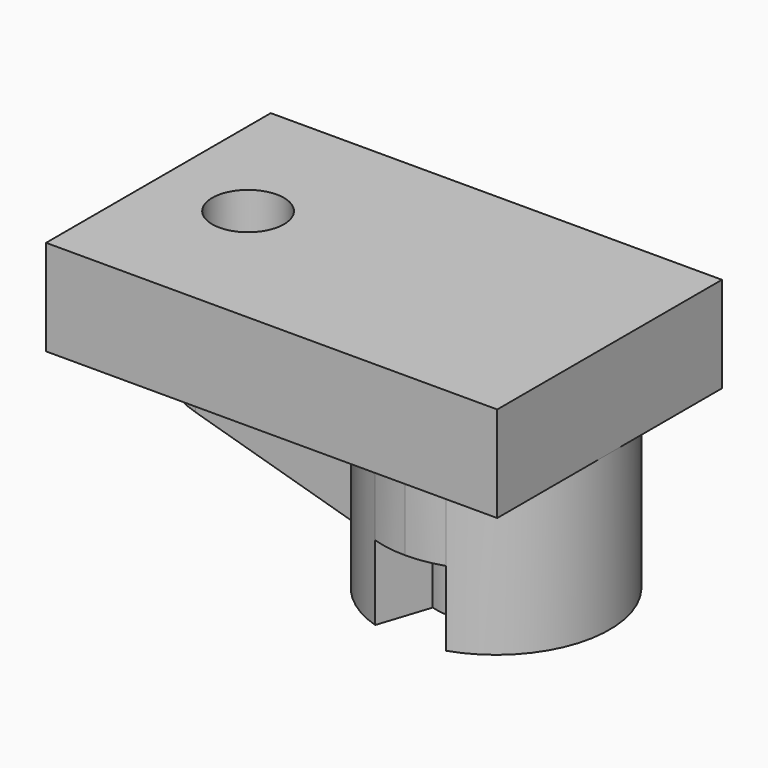
from build123d import *

# Parameters (mm, degrees)
F0_R      = 12
F1_DEPTH  = 32
F2_DEPTH  = 12
F3_DEPTH  = 52
F5_DEPTH  = 44
F6_DEPTH  = 93.7
F7_R      = 12
F8_DEPTH  = 98.4
F9_DEPTH  = 52
F11_DEPTH = 25


# Not quite as in the source:
# - a feature names something its author has since deleted; it is built from what else it names


with BuildPart() as f1:
    # F0 (on Top) → F1 (new body)
    with BuildSketch(Plane.XY):
        with BuildLine():
            Line((35.3547130823, 81.2151380405), (-47.6452869177, 81.2151380405))
            Line((-47.6452869177, 81.2151380405), (-47.6452869177, 56.2151380405))
            Line((-47.6452869177, 56.2151380405), (4.3708463127, 56.2151380405))
            ThreePointArc((4.3708463127, 56.2151380405), (13.0601260183, 64.9877132925), (24.1033321201, 70.5112318584))
            ThreePointArc((24.1033321201, 70.5112318584), (29.6648785101, 71.7867467702), (35.3547130823, 72.2151380405))
            Line((35.3547130823, 72.2151380405), (35.3547130823, 81.2151380405))
        make_face()
        with BuildLine():
            Line((-47.6452869177, 81.2151380405), (-77.6452869177, 81.2151380405))
            Line((-77.6452869177, 81.2151380405), (-77.6452869177, -12.7848619595))
            Line((-77.6452869177, -12.7848619595), (-47.6452869177, -12.7848619595))
            Line((-47.6452869177, -12.7848619595), (35.3547130823, -12.7848619595))
            Line((35.3547130823, -12.7848619595), (35.3547130823, -3.7848619595))
            ThreePointArc((35.3547130823, -3.7848619595), (29.5441458382, -3.3379884379), (23.8702411544, -2.0078781859))
            ThreePointArc((23.8702411544, -2.0078781859), (12.9613324626, 3.5143806488), (4.3708463127, 12.2151380405))
            Line((4.3708463127, 12.2151380405), (-47.6452869177, 12.2151380405))
            ThreePointArc((-47.6452869177, 12.2151380405), (-69.6452869177, 34.2151380405), (-47.6452869177, 56.2151380405))
            Line((-47.6452869177, 56.2151380405), (-47.6452869177, 81.2151380405))
        make_face()
        with BuildLine():
            Line((4.3708463127, 56.2151380405), (-47.6452869177, 56.2151380405))
            ThreePointArc((-47.6452869177, 56.2151380405), (-32.0889377316, 49.7714872266), (-25.6452869177, 34.2151380405))
            Line((-25.6452869177, 34.2151380405), (-2.6452869177, 34.2151380405))
            ThreePointArc((-2.6452869177, 34.2151380405), (-0.8487876963, 45.7609828072), (4.3708463127, 56.2151380405))
        make_face()
        with BuildLine():
            Line((-2.6452869177, 34.2151380405), (-25.6452869177, 34.2151380405))
            ThreePointArc((-25.6452869177, 34.2151380405), (-32.0889377316, 18.6587888544), (-47.6452869177, 12.2151380405))
            Line((-47.6452869177, 12.2151380405), (4.3708463127, 12.2151380405))
            ThreePointArc((4.3708463127, 12.2151380405), (-0.8487876963, 22.6692932738), (-2.6452869177, 34.2151380405))
        make_face()
        with BuildLine():
            ThreePointArc((-25.6452869177, 34.2151380405), (-32.0889377316, 49.7714872266), (-47.6452869177, 56.2151380405))
            ThreePointArc((-47.6452869177, 56.2151380405), (-69.6452869177, 34.2151380405), (-47.6452869177, 12.2151380405))
            ThreePointArc((-47.6452869177, 12.2151380405), (-32.0889377316, 18.6587888544), (-25.6452869177, 34.2151380405))
        make_face()
        with Locations((-47.6452869177, 34.2151380405)):
            Circle(F0_R, mode=Mode.SUBTRACT)
        with Locations((-47.6452869177, 34.2151380405)):
            Circle(F0_R)
        with BuildLine():
            ThreePointArc((24.1033321201, 70.5112318584), (13.0601260183, 64.9877132925), (4.3708463127, 56.2151380405))
            ThreePointArc((4.3708463127, 56.2151380405), (-0.8487876963, 45.7609828072), (-2.6452869177, 34.2151380405))
            ThreePointArc((-2.6452869177, 34.2151380405), (-0.8487876963, 22.6692932738), (4.3708463127, 12.2151380405))
            ThreePointArc((4.3708463127, 12.2151380405), (12.9613324626, 3.5143806488), (23.8702411544, -2.0078781859))
            Line((23.8702411544, -2.0078781859), (29.4328161154, 15.111967196))
            ThreePointArc((29.4328161154, 15.111967196), (32.3600024861, 14.440616341), (35.3547130823, 14.2151380405))
            Line((35.3547130823, 14.2151380405), (35.3547130823, 54.2151380405))
            ThreePointArc((35.3547130823, 54.2151380405), (32.4808372386, 54.0075819935), (29.6666104259, 53.389221804))
            Line((29.6666104259, 53.389221804), (24.1033321201, 70.5112318584))
        make_face()
        with BuildLine():
            ThreePointArc((47.4336065252, -1.8140214445), (66.2010901048, 12.0227739351), (73.3547130823, 34.2151380405))
            ThreePointArc((73.3547130823, 34.2151380405), (66.1022036315, 56.5443078622), (47.1130380862, 70.3501874123))
            Line((47.1130380862, 70.3501874123), (41.5507311927, 53.2311670575))
            ThreePointArc((41.5507311927, 53.2311670575), (38.4915442588, 53.9676135858), (35.3547130823, 54.2151380405))
            Line((35.3547130823, 54.2151380405), (35.3547130823, 14.2151380405))
            ThreePointArc((35.3547130823, 14.2151380405), (38.6581508077, 14.4898421189), (41.8708417514, 15.306408121))
            Line((41.8708417514, 15.306408121), (47.4336065252, -1.8140214445))
        make_face()
        with BuildLine():
            Line((73.3547130823, 81.2151380405), (35.3547130823, 81.2151380405))
            Line((35.3547130823, 81.2151380405), (35.3547130823, 72.2151380405))
            ThreePointArc((35.3547130823, 72.2151380405), (41.3073647549, 71.7460045115), (47.1130380862, 70.3501874123))
            ThreePointArc((47.1130380862, 70.3501874123), (66.1022036315, 56.5443078622), (73.3547130823, 34.2151380405))
            Line((73.3547130823, 34.2151380405), (73.3547130823, 81.2151380405))
        make_face()
        with BuildLine():
            Line((35.3547130823, 14.2151380405), (35.3547130823, -3.7848619595))
            ThreePointArc((35.3547130823, -3.7848619595), (41.4740243005, -3.2889154766), (47.4336065252, -1.8140214445))
            Line((47.4336065252, -1.8140214445), (41.8708417514, 15.306408121))
            ThreePointArc((41.8708417514, 15.306408121), (38.6581508077, 14.4898421189), (35.3547130823, 14.2151380405))
        make_face()
        with BuildLine():
            ThreePointArc((23.8702411544, -2.0078781859), (29.5441458382, -3.3379884379), (35.3547130823, -3.7848619595))
            Line((35.3547130823, -3.7848619595), (35.3547130823, 14.2151380405))
            ThreePointArc((35.3547130823, 14.2151380405), (32.3600024861, 14.440616341), (29.4328161154, 15.111967196))
            Line((29.4328161154, 15.111967196), (23.8702411544, -2.0078781859))
        make_face()
        with BuildLine():
            Line((35.3547130823, 54.2151380405), (35.3547130823, 72.2151380405))
            ThreePointArc((35.3547130823, 72.2151380405), (29.6648785101, 71.7867467702), (24.1033321201, 70.5112318584))
            Line((24.1033321201, 70.5112318584), (29.6666104259, 53.389221804))
            ThreePointArc((29.6666104259, 53.389221804), (32.4808372386, 54.0075819935), (35.3547130823, 54.2151380405))
        make_face()
        with BuildLine():
            ThreePointArc((47.1130380862, 70.3501874123), (41.3073647549, 71.7460045115), (35.3547130823, 72.2151380405))
            Line((35.3547130823, 72.2151380405), (35.3547130823, 54.2151380405))
            ThreePointArc((35.3547130823, 54.2151380405), (38.4915442588, 53.9676135858), (41.5507311927, 53.2311670575))
            Line((41.5507311927, 53.2311670575), (47.1130380862, 70.3501874123))
        make_face()
        with BuildLine():
            Line((35.3547130823, -3.7848619595), (35.3547130823, -12.7848619595))
            Line((35.3547130823, -12.7848619595), (73.3547130823, -12.7848619595))
            Line((73.3547130823, -12.7848619595), (73.3547130823, 34.2151380405))
            ThreePointArc((73.3547130823, 34.2151380405), (66.2010901048, 12.0227739351), (47.4336065252, -1.8140214445))
            ThreePointArc((47.4336065252, -1.8140214445), (41.4740243005, -3.2889154766), (35.3547130823, -3.7848619595))
        make_face()
    extrude(amount=F1_DEPTH)

    # F0 (on Top) → F2 (join)
    with BuildSketch(Plane.XY):
        with BuildLine():
            ThreePointArc((-25.6452869177, 34.2151380405), (-32.0889377316, 49.7714872266), (-47.6452869177, 56.2151380405))
            ThreePointArc((-47.6452869177, 56.2151380405), (-69.6452869177, 34.2151380405), (-47.6452869177, 12.2151380405))
            ThreePointArc((-47.6452869177, 12.2151380405), (-32.0889377316, 18.6587888544), (-25.6452869177, 34.2151380405))
        make_face()
        with Locations((-47.6452869177, 34.2151380405)):
            Circle(F0_R, mode=Mode.SUBTRACT)
        with BuildLine():
            Line((-2.6452869177, 34.2151380405), (-25.6452869177, 34.2151380405))
            ThreePointArc((-25.6452869177, 34.2151380405), (-32.0889377316, 18.6587888544), (-47.6452869177, 12.2151380405))
            Line((-47.6452869177, 12.2151380405), (4.3708463127, 12.2151380405))
            ThreePointArc((4.3708463127, 12.2151380405), (-0.8487876963, 22.6692932738), (-2.6452869177, 34.2151380405))
        make_face()
        with BuildLine():
            Line((4.3708463127, 56.2151380405), (-47.6452869177, 56.2151380405))
            ThreePointArc((-47.6452869177, 56.2151380405), (-32.0889377316, 49.7714872266), (-25.6452869177, 34.2151380405))
            Line((-25.6452869177, 34.2151380405), (-2.6452869177, 34.2151380405))
            ThreePointArc((-2.6452869177, 34.2151380405), (-0.8487876963, 45.7609828072), (4.3708463127, 56.2151380405))
        make_face()
    extrude(amount=-F2_DEPTH)

    # F0 (on Top) → F3 (join)
    with BuildSketch(Plane.XY):
        with BuildLine():
            ThreePointArc((47.4336065252, -1.8140214445), (66.2010901048, 12.0227739351), (73.3547130823, 34.2151380405))
            ThreePointArc((73.3547130823, 34.2151380405), (66.1022036315, 56.5443078622), (47.1130380862, 70.3501874123))
            Line((47.1130380862, 70.3501874123), (41.5507311927, 53.2311670575))
            ThreePointArc((41.5507311927, 53.2311670575), (38.4915442588, 53.9676135858), (35.3547130823, 54.2151380405))
            Line((35.3547130823, 54.2151380405), (35.3547130823, 14.2151380405))
            ThreePointArc((35.3547130823, 14.2151380405), (38.6581508077, 14.4898421189), (41.8708417514, 15.306408121))
            Line((41.8708417514, 15.306408121), (47.4336065252, -1.8140214445))
        make_face()
        with BuildLine():
            ThreePointArc((24.1033321201, 70.5112318584), (13.0601260183, 64.9877132925), (4.3708463127, 56.2151380405))
            ThreePointArc((4.3708463127, 56.2151380405), (-0.8487876963, 45.7609828072), (-2.6452869177, 34.2151380405))
            ThreePointArc((-2.6452869177, 34.2151380405), (-0.8487876963, 22.6692932738), (4.3708463127, 12.2151380405))
            ThreePointArc((4.3708463127, 12.2151380405), (12.9613324626, 3.5143806488), (23.8702411544, -2.0078781859))
            Line((23.8702411544, -2.0078781859), (29.4328161154, 15.111967196))
            ThreePointArc((29.4328161154, 15.111967196), (32.3600024861, 14.440616341), (35.3547130823, 14.2151380405))
            Line((35.3547130823, 14.2151380405), (35.3547130823, 54.2151380405))
            ThreePointArc((35.3547130823, 54.2151380405), (32.4808372386, 54.0075819935), (29.6666104259, 53.389221804))
            Line((29.6666104259, 53.389221804), (24.1033321201, 70.5112318584))
        make_face()
    extrude(amount=-F3_DEPTH)

    # F4 (on face) → F5 (join)
    with BuildSketch(Plane.XZ.offset(-12.2151380405)):
        Polygon((-47.6452869177, -12), (-69.6452869177, -12), (4.3708463127, -33.2237846755), (4.3708463127, -12), align=None)
    extrude(amount=-F5_DEPTH)

    # F6 (cut): faces of the model
    f6_faces = [f1.faces().sort_by_distance(p)[0] for p in [
        (-64.7311922609, 51.3010433837, -12),
        (-64.7311922609, 17.1292326973, -12),
    ]]
    extrude(f6_faces, amount=-F6_DEPTH, mode=Mode.SUBTRACT)

    # F7 (on face) → F8 (cut)
    with BuildSketch(Plane.XY.offset(32)):
        with Locations((-47.6452869177, 34.2151380405)):
            Circle(F7_R)
    extrude(amount=-F8_DEPTH, mode=Mode.SUBTRACT)

    # F0 (on Top) → F9 (join)
    with BuildSketch(Plane.XY):
        with BuildLine():
            ThreePointArc((47.1130380862, 70.3501874123), (41.3073647549, 71.7460045115), (35.3547130823, 72.2151380405))
            Line((35.3547130823, 72.2151380405), (35.3547130823, 54.2151380405))
            ThreePointArc((35.3547130823, 54.2151380405), (38.4915442588, 53.9676135858), (41.5507311927, 53.2311670575))
            Line((41.5507311927, 53.2311670575), (47.1130380862, 70.3501874123))
        make_face()
        with BuildLine():
            Line((35.3547130823, 54.2151380405), (35.3547130823, 72.2151380405))
            ThreePointArc((35.3547130823, 72.2151380405), (29.6648785101, 71.7867467702), (24.1033321201, 70.5112318584))
            Line((24.1033321201, 70.5112318584), (29.6666104259, 53.389221804))
            ThreePointArc((29.6666104259, 53.389221804), (32.4808372386, 54.0075819935), (35.3547130823, 54.2151380405))
        make_face()
        with BuildLine():
            Line((35.3547130823, 14.2151380405), (35.3547130823, -3.7848619595))
            ThreePointArc((35.3547130823, -3.7848619595), (41.4740243005, -3.2889154766), (47.4336065252, -1.8140214445))
            Line((47.4336065252, -1.8140214445), (41.8708417514, 15.306408121))
            ThreePointArc((41.8708417514, 15.306408121), (38.6581508077, 14.4898421189), (35.3547130823, 14.2151380405))
        make_face()
        with BuildLine():
            ThreePointArc((23.8702411544, -2.0078781859), (29.5441458382, -3.3379884379), (35.3547130823, -3.7848619595))
            Line((35.3547130823, -3.7848619595), (35.3547130823, 14.2151380405))
            ThreePointArc((35.3547130823, 14.2151380405), (32.3600024861, 14.440616341), (29.4328161154, 15.111967196))
            Line((29.4328161154, 15.111967196), (23.8702411544, -2.0078781859))
        make_face()
    extrude(amount=-F9_DEPTH)

    # F10 (on face) → F11 (cut)
    with BuildSketch(Plane(origin=(0, 0, -52), x_dir=(1, 0, 0), z_dir=(0, 0, -1))):
        with BuildLine():
            ThreePointArc((24.1033321201, -70.5112318584), (35.620667766, -72.2142073463), (47.1130380862, -70.3501874123))
            Line((47.1130380862, -70.3501874123), (41.5507311927, -53.2311670575))
            ThreePointArc((41.5507311927, -53.2311670575), (35.6206827287, -54.213369466), (29.6666104259, -53.389221804))
            Line((29.6666104259, -53.389221804), (24.1033321201, -70.5112318584))
        make_face()
        with BuildLine():
            ThreePointArc((29.4328161154, -15.111967196), (35.667330496, -14.2175814309), (41.8708417514, -15.306408121))
            Line((41.8708417514, -15.306408121), (47.4336065252, 1.8140214445))
            ThreePointArc((47.4336065252, 1.8140214445), (35.6673300099, 3.7835760253), (23.8702411544, 2.0078781859))
            Line((23.8702411544, 2.0078781859), (29.4328161154, -15.111967196))
        make_face()
    extrude(amount=-F11_DEPTH, mode=Mode.SUBTRACT)


solid = f1.part
